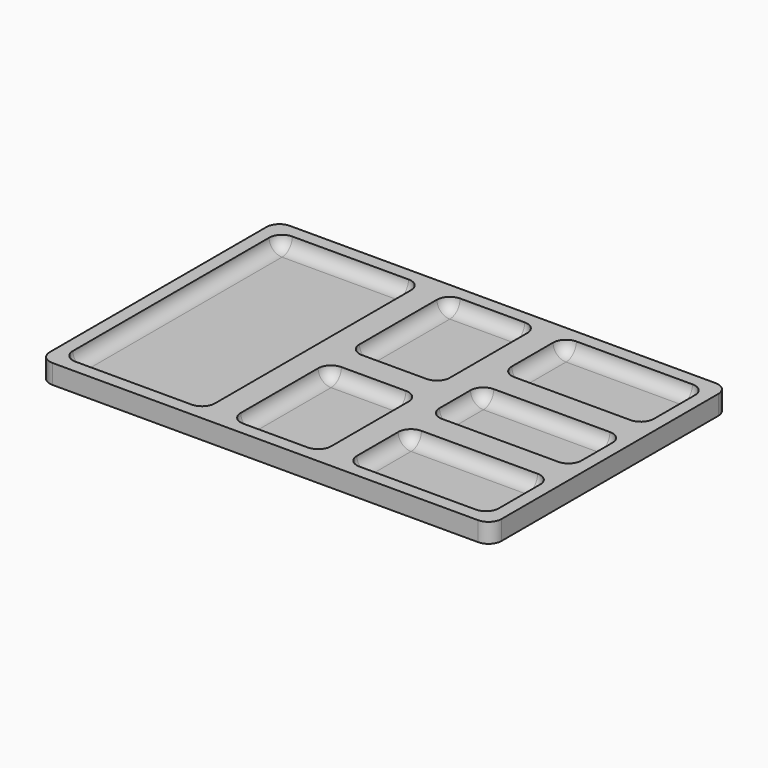
from build123d import *

# Parameters (mm, degrees)
F0_W     = 222.25
F0_H     = 146.05
F1_DEPTH = 9.525
F2_W     = 69.85
F2_H     = 38.1
F2_H_2   = 133.35
F2_H_3   = 31.75
F2_W_2   = 44.45
F2_H_4   = 60.325
F3_DEPTH = 6.35
F4_F1_R  = 6.35
F4_F2_R  = 6.35
F4_F3_R  = 6.35
F4_F4_R  = 6.35
F4_F5_R  = 6.35
F4_F6_R  = 6.3499
F4_F7_R  = 6.35
F4_F8_R  = 6.3499
F4_F9_R  = 6.35
F4_F10_R = 6.35
F4_F11_R = 6.3499
F4_F12_R = 6.3499
F4_F13_R = 6.35
F4_F14_R = 6.3499
F4_F15_R = 6.3499
F4_F16_R = 6.3499
F4_F17_R = 6.35
F4_F18_R = 6.35
F4_F19_R = 6.3499
F4_F20_R = 6.3499
F4_F21_R = 6.35
F4_F22_R = 6.3499
F4_F23_R = 6.3499
F4_F24_R = 6.3499
F4_F25_R = 6.35
F4_F26_R = 6.35
F4_F27_R = 6.3499
F4_F28_R = 6.3499


# Not quite as in the source:
# - two fillets or chamfers of one size are made in one step
# - a fillet or chamfer is up to 0.001 mm smaller than in the source, because OpenCascade refuses the exact size
# - a feature of the source that left no trace in its solid (it failed there, or was rolled back) is left out


with BuildPart() as f1:
    # F0 (on Top) → F1 (new body)
    with BuildSketch(Plane.XY):
        Rectangle(F0_W, F0_H)
    extrude(amount=F1_DEPTH)

    # F2 (on face) → F3 (cut)
    with BuildSketch(Plane.XY.offset(9.525)):
        with Locations((69.85, 47.625)):
            Rectangle(F2_W, F2_H)
        with Locations((69.85, -47.625)):
            Rectangle(F2_W, F2_H)
        with Locations((-69.85, 0)):
            Rectangle(F2_W, F2_H_2)
        with Locations((69.85, 0)):
            Rectangle(F2_W, F2_H_3)
        with Locations((0, -36.5125)):
            Rectangle(F2_W_2, F2_H_4)
        with Locations((0, 36.5125)):
            Rectangle(F2_W_2, F2_H_4)
    extrude(amount=-F3_DEPTH, mode=Mode.SUBTRACT)

    # F4: fillet of radius 6.35 on 46 edges, made by hand

    # F4_f1
    f4_f1_edges = [f1.edges().sort_by_distance(p)[0] for p in [
        (111.125, -73.025, 4.7625),
    ]]
    fillet(f4_f1_edges, radius=F4_F1_R)

    # F4_f2
    f4_f2_edges = [f1.edges().sort_by_distance(p)[0] for p in [
        (111.125, 73.025, 4.7625),
    ]]
    fillet(f4_f2_edges, radius=F4_F2_R)

    # F4_f3
    f4_f3_edges = [f1.edges().sort_by_distance(p)[0] for p in [
        (-111.125, -73.025, 4.7625),
    ]]
    fillet(f4_f3_edges, radius=F4_F3_R)

    # F4_f4
    f4_f4_edges = [f1.edges().sort_by_distance(p)[0] for p in [
        (-111.125, 73.025, 4.7625),
    ]]
    fillet(f4_f4_edges, radius=F4_F4_R)

    # F4_f5
    f4_f5_edges = [f1.edges().sort_by_distance(p)[0] for p in [
        (-22.225, -6.35, 6.35),
    ]]
    fillet(f4_f5_edges, radius=F4_F5_R)

    # F4_f6 (radius 6.35 in the source; OpenCascade refuses exactly that, so slightly less here)
    f4_f6_edges = [f1.edges().sort_by_distance(p)[0] for p in [
        (-22.225, -39.6875, 3.175),
    ]]
    fillet(f4_f6_edges, radius=F4_F6_R)

    # F4_f7
    f4_f7_edges = [f1.edges().sort_by_distance(p)[0] for p in [
        (22.225, -66.675, 6.35),
    ]]
    fillet(f4_f7_edges, radius=F4_F7_R)

    # F4_f8 (radius 6.35 in the source; OpenCascade refuses exactly that, so slightly less here)
    f4_f8_edges = [f1.edges().sort_by_distance(p)[0] for p in [
        (-5e-05, -66.675, 3.175),
    ]]
    fillet(f4_f8_edges, radius=F4_F8_R)

    # F4_f9
    f4_f9_edges = [f1.edges().sort_by_distance(p)[0] for p in [
        (34.925, -66.675, 6.35),
    ]]
    fillet(f4_f9_edges, radius=F4_F9_R)

    # F4_f10
    f4_f10_edges = [f1.edges().sort_by_distance(p)[0] for p in [
        (104.775, -66.675, 6.35),
    ]]
    fillet(f4_f10_edges, radius=F4_F10_R)

    # F4_f11 (radius 6.35 in the source; OpenCascade refuses exactly that, so slightly less here)
    f4_f11_edges = [f1.edges().sort_by_distance(p)[0] for p in [
        (69.85, -66.675, 3.175),
    ]]
    fillet(f4_f11_edges, radius=F4_F11_R)

    # F4_f12 (radius 6.35 in the source; OpenCascade refuses exactly that, so slightly less here)
    f4_f12_edges = [f1.edges().sort_by_distance(p)[0] for p in [
        (104.775, -28.575, 9.52495),
    ]]
    fillet(f4_f12_edges, radius=F4_F12_R)

    # F4_f13
    f4_f13_edges = [f1.edges().sort_by_distance(p)[0] for p in [
        (-34.925, 66.675, 6.35),
    ]]
    fillet(f4_f13_edges, radius=F4_F13_R)

    # F4_f14 (radius 6.35 in the source; OpenCascade refuses exactly that, so slightly less here)
    f4_f14_edges = [f1.edges().sort_by_distance(p)[0] for p in [
        (-73.025, 66.675, 3.175),
    ]]
    fillet(f4_f14_edges, radius=F4_F14_R)

    # F4_f15 (radius 6.35 in the source; OpenCascade refuses exactly that, so slightly less here)
    f4_f15_edges = [f1.edges().sort_by_distance(p)[0] for p in [
        (-104.775, -3.17495, 3.175),
    ]]
    fillet(f4_f15_edges, radius=F4_F15_R)

    # F4_f16 (radius 6.35 in the source; OpenCascade refuses exactly that, so slightly less here)
    f4_f16_edges = [f1.edges().sort_by_distance(p)[0] for p in [
        (-34.925, -66.675, 9.52495),
    ]]
    fillet(f4_f16_edges, radius=F4_F16_R)

    # F4_f17
    f4_f17_edges = [f1.edges().sort_by_distance(p)[0] for p in [
        (104.775, -15.875, 6.35),
    ]]
    fillet(f4_f17_edges, radius=F4_F17_R)

    # F4_f18
    f4_f18_edges = [f1.edges().sort_by_distance(p)[0] for p in [
        (104.775, 15.875, 6.35),
    ]]
    fillet(f4_f18_edges, radius=F4_F18_R)

    # F4_f19 (radius 6.35 in the source; OpenCascade refuses exactly that, so slightly less here)
    f4_f19_edges = [f1.edges().sort_by_distance(p)[0] for p in [
        (104.775, 0, 3.175),
    ]]
    fillet(f4_f19_edges, radius=F4_F19_R)

    # F4_f20 (radius 6.35 in the source; OpenCascade refuses exactly that, so slightly less here)
    f4_f20_edges = [f1.edges().sort_by_distance(p)[0] for p in [
        (34.925, 15.875, 9.52495),
    ]]
    fillet(f4_f20_edges, radius=F4_F20_R)

    # F4_f21
    f4_f21_edges = [f1.edges().sort_by_distance(p)[0] for p in [
        (22.225, 6.35, 6.35),
    ]]
    fillet(f4_f21_edges, radius=F4_F21_R)

    # F4_f22 (radius 6.35 in the source; OpenCascade refuses exactly that, so slightly less here)
    f4_f22_edges = [f1.edges().sort_by_distance(p)[0] for p in [
        (22.225, 39.6875, 3.175),
    ]]
    fillet(f4_f22_edges, radius=F4_F22_R)

    # F4_f23 (radius 6.35 in the source; OpenCascade refuses exactly that, so slightly less here)
    f4_f23_edges = [f1.edges().sort_by_distance(p)[0] for p in [
        (-3.17495, 66.675, 3.175),
    ]]
    fillet(f4_f23_edges, radius=F4_F23_R)

    # F4_f24 (radius 6.35 in the source; OpenCascade refuses exactly that, so slightly less here)
    f4_f24_edges = [f1.edges().sort_by_distance(p)[0] for p in [
        (-22.225, 6.35, 9.52495),
    ]]
    fillet(f4_f24_edges, radius=F4_F24_R)

    # F4_f25
    f4_f25_edges = [f1.edges().sort_by_distance(p)[0] for p in [
        (104.775, 28.575, 6.35),
    ]]
    fillet(f4_f25_edges, radius=F4_F25_R)

    # F4_f26
    f4_f26_edges = [f1.edges().sort_by_distance(p)[0] for p in [
        (104.775, 66.675, 6.35),
    ]]
    fillet(f4_f26_edges, radius=F4_F26_R)

    # F4_f27 (radius 6.35 in the source; OpenCascade refuses exactly that, so slightly less here)
    f4_f27_edges = [f1.edges().sort_by_distance(p)[0] for p in [
        (104.775, 47.625, 3.175),
    ]]
    fillet(f4_f27_edges, radius=F4_F27_R)

    # F4_f28 (radius 6.35 in the source; OpenCascade refuses exactly that, so slightly less here)
    f4_f28_edges = [f1.edges().sort_by_distance(p)[0] for p in [
        (34.925, 66.675, 9.52495),
    ]]
    fillet(f4_f28_edges, radius=F4_F28_R)


solid = f1.part
